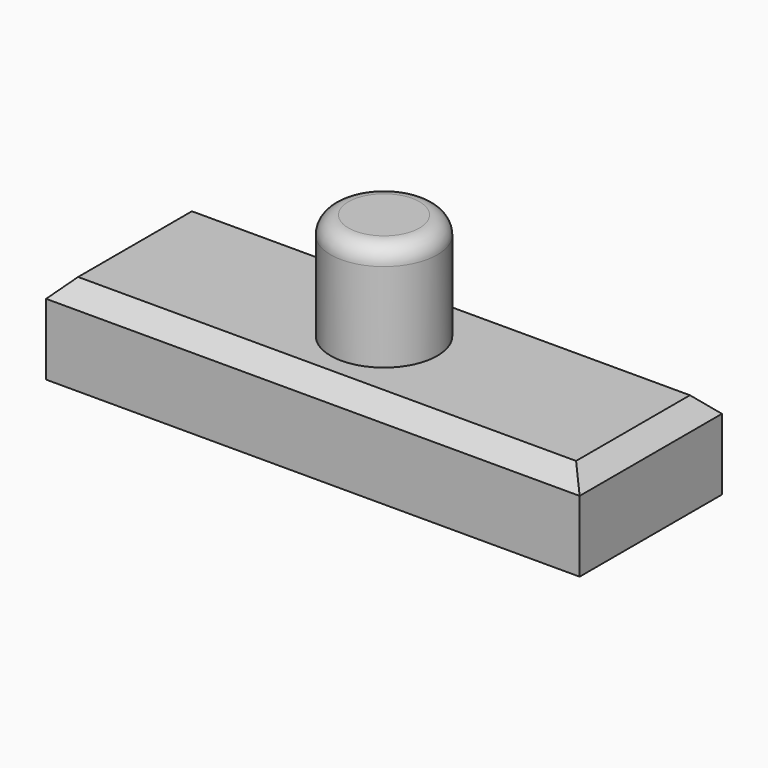
from build123d import *

# Parameters (mm, degrees)
F0_W     = 150
F0_H     = 50
F1_DEPTH = 25
F3_DEPTH = 30
F4_R     = 5
F5_SIZE  = 5


with BuildPart() as f1:
    # F0 (on Top) → F1 (new body)
    with BuildSketch(Plane.XY):
        with Locations((13.5704912245, -12.3678184533)):
            Rectangle(F0_W, F0_H)
    extrude(amount=F1_DEPTH)

    # F2 (on face) → F3 (join)
    with BuildSketch(Plane.XY.offset(25)):
        with BuildLine():
            Line((-1.4295087755, -12.3678184533), (28.5704912245, -12.3678184533))
            ThreePointArc((28.5704912245, -12.3678184533), (13.5704912245, 2.6321815467), (-1.4295087755, -12.3678184533))
        make_face()
        with BuildLine():
            ThreePointArc((-1.4295087755, -12.3678184533), (13.5704912245, -27.3678184533), (28.5704912245, -12.3678184533))
            Line((28.5704912245, -12.3678184533), (-1.4295087755, -12.3678184533))
        make_face()
    extrude(amount=F3_DEPTH)

    # F4
    f4_edges = [f1.edges().sort_by_distance(p)[0] for p in [
        (28.570491, -12.367818, 55),
    ]]
    fillet(f4_edges, radius=F4_R)

    # F5
    f5_edges = [f1.edges().sort_by_distance(p)[0] for p in [
        (-61.429509, -12.367818, 25),
        (13.570491, -37.367818, 25),
        (13.570491, 12.632182, 25),
        (88.570491, -12.367818, 25),
    ]]
    chamfer(f5_edges, length=F5_SIZE)


solid = f1.part
